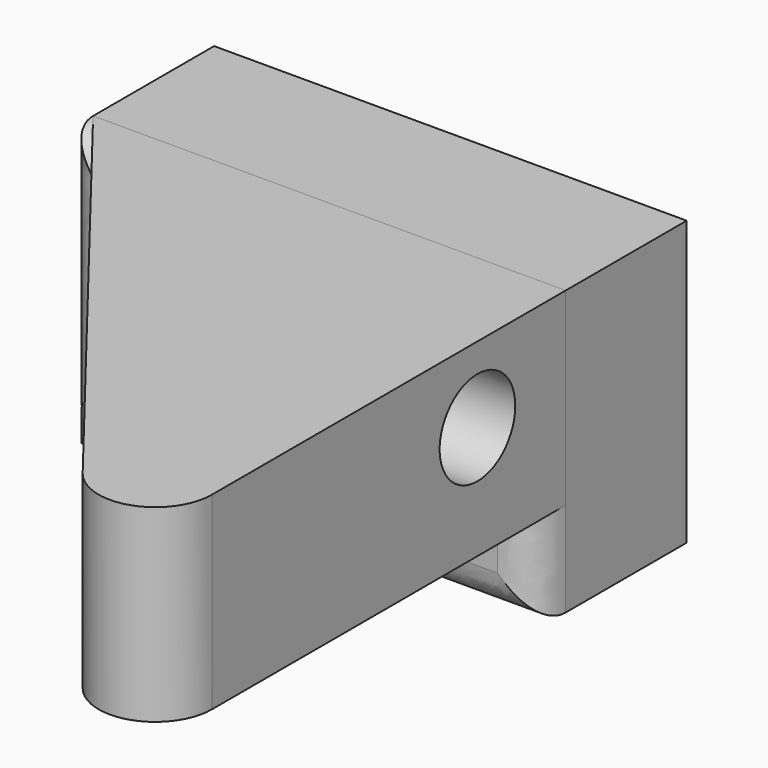
from build123d import *

# Parameters (mm, degrees)
F0_W        = 63.5
F0_H        = 38.1
F1_DEPTH    = 25.4
F2_T1_DEPTH = 63.5
F2_T3_DEPTH = 88.9
F4_DEPTH    = 25.399999693
F5_R        = 6.35
F6_DEPTH    = 56.9109635576
F7_R        = 7.62


# Not quite as in the source:
# - a fillet or chamfer that OpenCascade refuses, or shapes differently, is made with other operations: its cross-section is extruded or revolved along the edge and cut away or added


with BuildPart() as f1:
    # F0 (on Front) → F1 (new body)
    with BuildSketch(Plane.XZ):
        with Locations((31.75, 19.05)):
            Rectangle(F0_W, F0_H)
    extrude(amount=F1_DEPTH)

    # F2: fillet of radius 5.08 on 4 edges, made by hand

    # F2_s2 → F2_t1 (cut)
    with BuildSketch(Plane.XY.offset(-12.7)):
        with BuildLine():
            add(Edge.make_bspline(
                [(0, -20.32), (0, -25.4), (5.08, -25.4)],
                knots=[0, 0, 0, 1, 1, 1], degree=2, weights=[1, 0.8181818182, 1]))
            Line((5.08, -25.4), (0, -25.4))
            Line((0, -25.4), (0, -20.32))
        make_face()
        with BuildLine():
            add(Edge.make_bspline(
                [(63.5, -20.32), (63.5, -25.4), (58.42, -25.4)],
                knots=[0, 0, 0, 1, 1, 1], degree=2, weights=[1, 0.8181818182, 1]))
            Line((58.42, -25.4), (63.5, -25.4))
            Line((63.5, -25.4), (63.5, -20.32))
        make_face()
    extrude(amount=F2_T1_DEPTH, mode=Mode.SUBTRACT)

    # F2_s4 → F2_t3 (cut)
    with BuildSketch(Plane.YZ.offset(-12.7)):
        with BuildLine():
            add(Edge.make_bspline(
                [(-20.32, 0), (-25.4, 0), (-25.4, 5.08)],
                knots=[0, 0, 0, 1, 1, 1], degree=2, weights=[1, 0.8181818182, 1]))
            Line((-25.4, 5.08), (-25.4, 0))
            Line((-25.4, 0), (-20.32, 0))
        make_face()
        with BuildLine():
            add(Edge.make_bspline(
                [(-20.32, 38.1), (-25.4, 38.1), (-25.4, 33.02)],
                knots=[0, 0, 0, 1, 1, 1], degree=2, weights=[1, 0.8181818182, 1]))
            Line((-25.4, 33.02), (-25.4, 38.1))
            Line((-25.4, 38.1), (-20.32, 38.1))
        make_face()
    extrude(amount=F2_T3_DEPTH, mode=Mode.SUBTRACT)


with BuildPart() as f4:
    # F3 (on face) → F4 (new body)
    with BuildSketch(Plane.XY.offset(38.1)):
        Polygon((0, -20.32), (63.5, -101.9336432219), (63.5, -20.32), align=None)
    extrude(amount=-F4_DEPTH)

    # F5 (on face) → F6 (cut, through all)
    with BuildSketch(Plane.YZ.offset(63.5)):
        with Locations((-35.1398721737, 27.9031097638)):
            Circle(F5_R)
    extrude(amount=-F6_DEPTH, mode=Mode.SUBTRACT)

    # F7
    f7_edges = [f4.edges().sort_by_distance(p)[0] for p in [
        (63.5, -101.933643, 25.4),
    ]]
    fillet(f7_edges, radius=F7_R)


solid = Compound([f1.part, f4.part])
